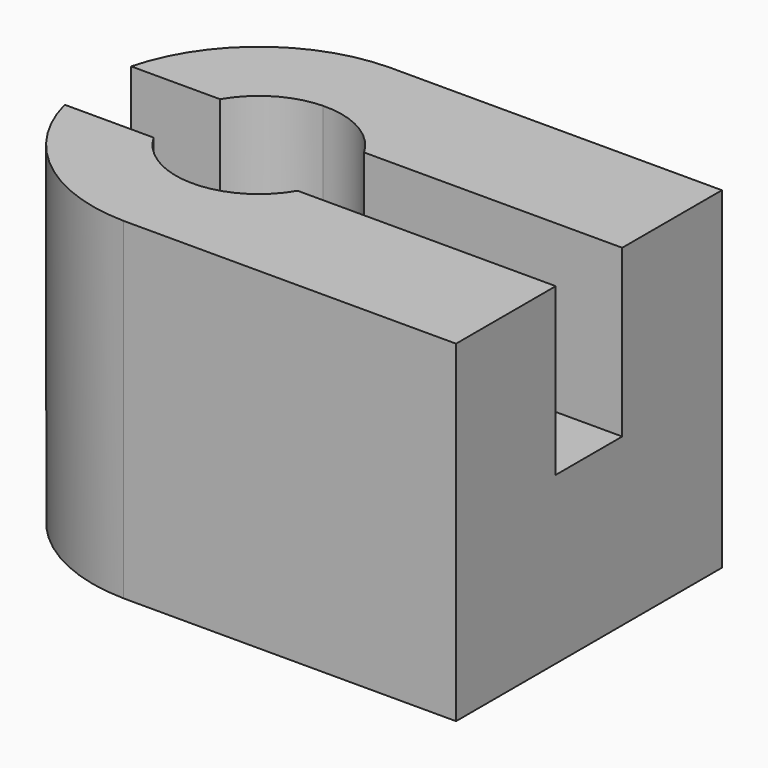
from build123d import *

# Parameters (mm, degrees)
F1_DEPTH = 20
F2_W     = 5
F2_H     = 10
F3_DEPTH = 29.868809509


with BuildPart() as f1:
    # F0 (on Top) → F1 (new body)
    with BuildSketch(Plane.XY):
        with BuildLine():
            ThreePointArc((-34.9428019347, -9.9991262455), (-27.7864355102, -7.117650768), (-24.8106114437, 0))
            ThreePointArc((-24.8106114437, 0), (-27.6929606757, 7.0241759335), (-34.6784209527, 9.9991262455))
            Line((-34.6784209527, 9.9991262455), (-34.9428019347, 9.9991262455))
            Line((-34.9428019347, 9.9991262455), (-34.9428019347, 4.998252262))
            ThreePointArc((-34.9428019347, 4.998252262), (-31.3221269916, 3.581965414), (-29.8106114437, 0))
            ThreePointArc((-29.8106114437, 0), (-31.3221269916, -3.581965414), (-34.9428019347, -4.998252262))
            Line((-34.9428019347, -4.998252262), (-34.9428019347, -9.9991262455))
        make_face()
        with BuildLine():
            ThreePointArc((-34.6784209527, 9.9991262455), (-27.6929606757, 7.0241759335), (-24.8106114437, 0))
            ThreePointArc((-24.8106114437, 0), (-27.7864355102, -7.117650768), (-34.9428019347, -9.9991262455))
            Line((-34.9428019347, -9.9991262455), (-34.9428019347, -10.0008737545))
            Line((-34.9428019347, -10.0008737545), (-14.9428019347, -10.0008737545))
            Line((-14.9428019347, -10.0008737545), (-14.9428019347, 9.9991262455))
            Line((-14.9428019347, 9.9991262455), (-34.6784209527, 9.9991262455))
        make_face()
        with BuildLine():
            Line((-34.9428019347, 9.9991262455), (-34.6784209527, 9.9991262455))
            ThreePointArc((-34.6784209527, 9.9991262455), (-34.8106114437, 10), (-34.9428019347, 9.9991262455))
        make_face()
        with BuildLine():
            ThreePointArc((-34.9428019347, 9.9991262455), (-44.8106114437, 0), (-34.9428019347, -9.9991262455))
            Line((-34.9428019347, -9.9991262455), (-34.9428019347, -4.998252262))
            ThreePointArc((-34.9428019347, -4.998252262), (-39.8106114437, 0), (-34.9428019347, 4.998252262))
            Line((-34.9428019347, 4.998252262), (-34.9428019347, 9.9991262455))
        make_face()
    extrude(amount=F1_DEPTH)

    # F2 (on face) → F3 (cut, through all)
    with BuildSketch(Plane.YZ.offset(-14.9428019347)):
        with Locations((-0.0008737545, 15)):
            Rectangle(F2_W, F2_H)
    extrude(amount=-F3_DEPTH, mode=Mode.SUBTRACT)


solid = f1.part
